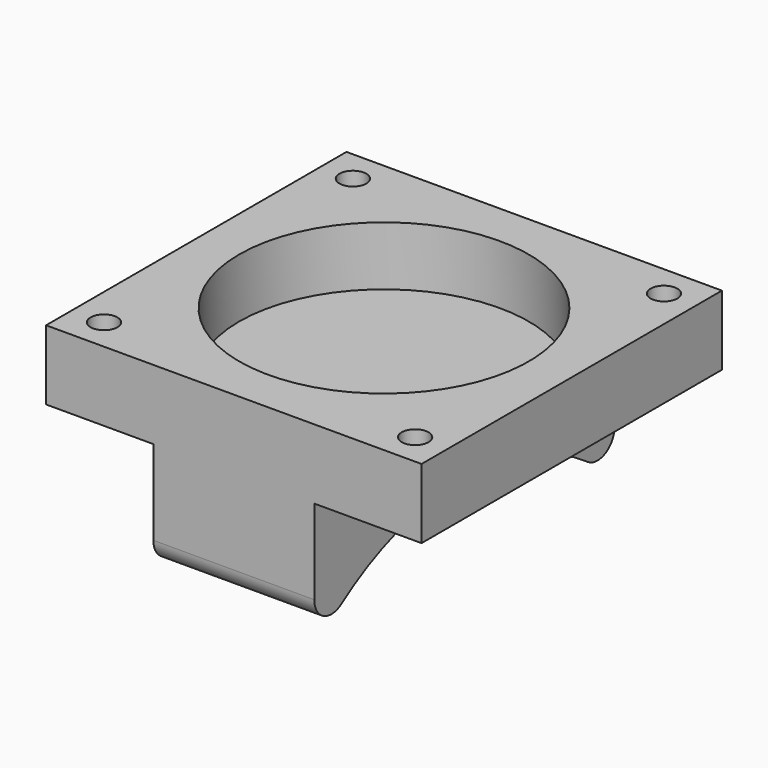
from build123d import *

# Parameters (mm, degrees)
F0_W       = 35
F0_H       = 35
F0_W_2     = 23
F0_H_2     = 23
F1_DEPTH   = 2
F3_DEPTH   = 5.5
F4_DEPTH   = 2.5
F5_DEPTH   = 1
F7_W       = 35
F7_H       = 35
F7_R       = 13.5
F8_DEPTH   = 1
F9_D       = 2.5
F9_DEPTH   = 10
F9_TIP     = 0.7510757738
F9_2_D     = 2.5
F9_2_DEPTH = 10
F9_2_TIP   = 0.7510757738
F10_W      = 7.5
F10_H      = 17.5
F11_DEPTH  = 25
F12_R      = 25
F13_DEPTH  = 25
F14_R      = 2


with BuildPart() as f1:
    # F0 (on Top) → F1 (new body)
    with BuildSketch(Plane.XY):
        with Locations((-9.5, 9.5)):
            Rectangle(F0_W, F0_H)
        with Locations((-9.5, 9.5)):
            Rectangle(F0_W_2, F0_H_2, mode=Mode.SUBTRACT)
        with Locations((-9.5, 9.5)):
            Rectangle(F0_W_2, F0_H_2)
        with BuildLine():
            Line((0, 5.027864045), (0, 0))
            Line((0, 0), (-5.027864045, 0))
            ThreePointArc((-5.027864045, 0), (-9.5, -1), (-13.972135955, 0))
            Line((-13.972135955, 0), (-19, 0))
            Line((-19, 0), (-19, 5.027864045))
            ThreePointArc((-19, 5.027864045), (-20, 9.5), (-19, 13.972135955))
            Line((-19, 13.972135955), (-19, 19))
            Line((-19, 19), (-13.972135955, 19))
            ThreePointArc((-13.972135955, 19), (-9.5, 20), (-5.027864045, 19))
            Line((-5.027864045, 19), (0, 19))
            Line((0, 19), (0, 13.972135955))
            ThreePointArc((0, 13.972135955), (0.746950766, 11.7912878475), (1, 9.5))
            ThreePointArc((1, 9.5), (0.746950766, 7.2087121525), (0, 5.027864045))
        make_face(mode=Mode.SUBTRACT)
        with BuildLine():
            Line((-13.972135955, 0), (-5.027864045, 0))
            ThreePointArc((-5.027864045, 0), (-2.0753787975, 2.0753787975), (0, 5.027864045))
            Line((0, 5.027864045), (0, 13.972135955))
            ThreePointArc((0, 13.972135955), (-2.0753787975, 16.9246212025), (-5.027864045, 19))
            Line((-5.027864045, 19), (-13.972135955, 19))
            ThreePointArc((-13.972135955, 19), (-16.9246212025, 16.9246212025), (-19, 13.972135955))
            Line((-19, 13.972135955), (-19, 5.027864045))
            ThreePointArc((-19, 5.027864045), (-16.9246212025, 2.0753787975), (-13.972135955, 0))
        make_face()
        with BuildLine():
            Line((-19, 19), (-19, 13.972135955))
            ThreePointArc((-19, 13.972135955), (-16.9246212025, 16.9246212025), (-13.972135955, 19))
            Line((-13.972135955, 19), (-19, 19))
        make_face()
        with BuildLine():
            ThreePointArc((-5.027864045, 19), (-2.0753787975, 16.9246212025), (0, 13.972135955))
            Line((0, 13.972135955), (0, 19))
            Line((0, 19), (-5.027864045, 19))
        make_face()
        with BuildLine():
            Line((-5.027864045, 0), (0, 0))
            Line((0, 0), (0, 5.027864045))
            ThreePointArc((0, 5.027864045), (-2.0753787975, 2.0753787975), (-5.027864045, 0))
        make_face()
        with BuildLine():
            Line((-19, 0), (-13.972135955, 0))
            ThreePointArc((-13.972135955, 0), (-16.9246212025, 2.0753787975), (-19, 5.027864045))
            Line((-19, 5.027864045), (-19, 0))
        make_face()
        with BuildLine():
            Line((0, 13.972135955), (0, 5.027864045))
            ThreePointArc((0, 5.027864045), (0.746950766, 7.2087121525), (1, 9.5))
            ThreePointArc((1, 9.5), (0.746950766, 11.7912878475), (0, 13.972135955))
        make_face()
        with BuildLine():
            ThreePointArc((-13.972135955, 0), (-9.5, -1), (-5.027864045, 0))
            Line((-5.027864045, 0), (-13.972135955, 0))
        make_face()
        with BuildLine():
            ThreePointArc((-19, 13.972135955), (-20, 9.5), (-19, 5.027864045))
            Line((-19, 5.027864045), (-19, 13.972135955))
        make_face()
        with BuildLine():
            Line((-13.972135955, 19), (-5.027864045, 19))
            ThreePointArc((-5.027864045, 19), (-9.5, 20), (-13.972135955, 19))
        make_face()
    extrude(amount=-F1_DEPTH)

    # F0 (on Top) → F4 (join)
    with BuildSketch(Plane.XY):
        with Locations((-9.5, 9.5)):
            Rectangle(F0_W_2, F0_H_2)
        with BuildLine():
            Line((0, 5.027864045), (0, 0))
            Line((0, 0), (-5.027864045, 0))
            ThreePointArc((-5.027864045, 0), (-9.5, -1), (-13.972135955, 0))
            Line((-13.972135955, 0), (-19, 0))
            Line((-19, 0), (-19, 5.027864045))
            ThreePointArc((-19, 5.027864045), (-20, 9.5), (-19, 13.972135955))
            Line((-19, 13.972135955), (-19, 19))
            Line((-19, 19), (-13.972135955, 19))
            ThreePointArc((-13.972135955, 19), (-9.5, 20), (-5.027864045, 19))
            Line((-5.027864045, 19), (0, 19))
            Line((0, 19), (0, 13.972135955))
            ThreePointArc((0, 13.972135955), (0.746950766, 11.7912878475), (1, 9.5))
            ThreePointArc((1, 9.5), (0.746950766, 7.2087121525), (0, 5.027864045))
        make_face(mode=Mode.SUBTRACT)
        with BuildLine():
            ThreePointArc((-19, 13.972135955), (-20, 9.5), (-19, 5.027864045))
            Line((-19, 5.027864045), (-19, 13.972135955))
        make_face()
        with BuildLine():
            Line((-13.972135955, 19), (-5.027864045, 19))
            ThreePointArc((-5.027864045, 19), (-9.5, 20), (-13.972135955, 19))
        make_face()
        with BuildLine():
            Line((0, 13.972135955), (0, 5.027864045))
            ThreePointArc((0, 5.027864045), (0.746950766, 7.2087121525), (1, 9.5))
            ThreePointArc((1, 9.5), (0.746950766, 11.7912878475), (0, 13.972135955))
        make_face()
        with BuildLine():
            ThreePointArc((-13.972135955, 0), (-9.5, -1), (-5.027864045, 0))
            Line((-5.027864045, 0), (-13.972135955, 0))
        make_face()
    extrude(amount=F4_DEPTH)


with BuildPart() as f3:
    # F2 (on face) → F3 (new body)
    with BuildSketch(Plane(origin=(0, 0, -2), x_dir=(1, 0, 0), z_dir=(0, 0, -1))):
        with BuildLine():
            Line((-27, -9.5), (-27, -27))
            Line((-27, -27), (8, -27))
            Line((8, -27), (8, -9.5))
            Line((8, -9.5), (4, -9.5))
            ThreePointArc((4, -9.5), (-9.5, -23), (-23, -9.5))
            Line((-23, -9.5), (-27, -9.5))
        make_face()
        with BuildLine():
            Line((-27, 8), (-27, -9.5))
            Line((-27, -9.5), (-23, -9.5))
            ThreePointArc((-23, -9.5), (-9.5, 4), (4, -9.5))
            Line((4, -9.5), (8, -9.5))
            Line((8, -9.5), (8, 8))
            Line((8, 8), (-27, 8))
        make_face()
    extrude(amount=F3_DEPTH)


with BuildPart() as f5:
    # F5 (new): a face of the model
    f5_faces = [f3.part.faces().sort_by_distance(p)[0] for p in [
        (-9.5, 26.5050252532, -7.5),
    ]]
    extrude(f5_faces, amount=F5_DEPTH)


with BuildPart() as f5b:
    # F5#2 (new): a face of the model
    f5_2_faces = [f1.part.faces().sort_by_distance(p)[0] for p in [
        (-9.5, 9.5, -2),
    ]]
    extrude(f5_2_faces, amount=F5_DEPTH)


with BuildPart() as f3_1:
    add(f3.part)

    # F7 (on face) → F8 (join)
    with BuildSketch(Plane(origin=(0, 0, -7.5), x_dir=(1, 0, 0), z_dir=(0, 0, -1))):
        with Locations((-9.5, -9.5)):
            Rectangle(F7_W, F7_H)
        with Locations((-9.5, -9.5)):
            Circle(F7_R, mode=Mode.SUBTRACT)
        with Locations((-9.5, -9.5)):
            Circle(F7_R)
    extrude(amount=F8_DEPTH)

    # F9#2
    with Locations(Plane.XY):
        with Locations((-24, -5), (-24, 24), (5, 24), (5, -5)):
            Hole(F9_2_D / 2, depth=F9_2_DEPTH)
            with Locations((0, 0, -(F9_2_DEPTH + F9_2_TIP / 2))):  # 118° drill point
                Cone(0, F9_2_D / 2, F9_2_TIP, mode=Mode.SUBTRACT)

    # F10 (on face) → F11 (join)
    with BuildSketch(Plane(origin=(0, 0, -8.5), x_dir=(1, 0, 0), z_dir=(0, 0, -1))):
        with Locations((-13.25, -0.75)):
            Rectangle(F10_W, F10_H)
        with Locations((-13.25, -18.25)):
            Rectangle(F10_W, F10_H)
        Polygon((-2, 8), (-9.5, 8), (-9.5, -9.5), (-9.5, -27), (-2, -27), (-2, -9.5), align=None)
    extrude(amount=F11_DEPTH)

    # F12 (on face) → F13 (cut)
    with BuildSketch(Plane(origin=(-17, 0, 0), x_dir=(0, -1, 0), z_dir=(-1, 0, 0))):
        with Locations((-9.5, -38.5)):
            Circle(F12_R)
    extrude(amount=-F13_DEPTH, mode=Mode.SUBTRACT)

    # F14
    f14_edges = [f3_1.edges().sort_by_distance(p)[0] for p in [
        (-9.5, -8, -20.646429),
        (-9.5, 27, -20.646429),
    ]]
    fillet(f14_edges, radius=F14_R)


with BuildPart() as f1_1:
    add(f1.part)

    # F9
    with Locations(Plane.XY):
        with Locations((-24, -5), (-24, 24), (5, 24), (5, -5)):
            Hole(F9_D / 2, depth=F9_DEPTH)
            with Locations((0, 0, -(F9_DEPTH + F9_TIP / 2))):  # 118° drill point
                Cone(0, F9_D / 2, F9_TIP, mode=Mode.SUBTRACT)


solid = f3_1.part
